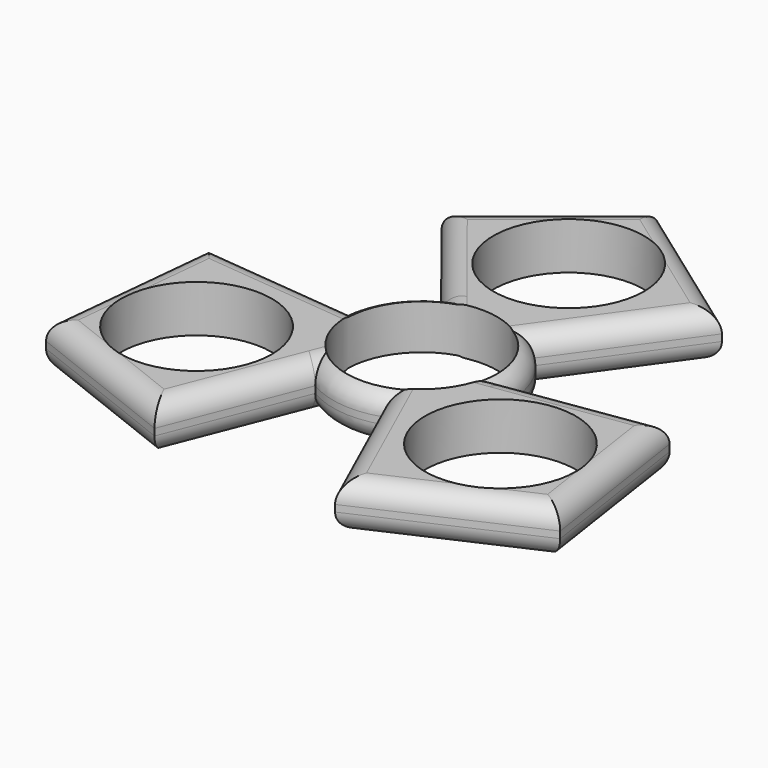
from build123d import *

# Parameters (mm, degrees)
F0_R          = 11.2
F1_DEPTH      = 7
F2_T1_DEPTH   = 41.9845753996
F2_T3_DEPTH   = 40.2947851744
F2_T5_DEPTH   = 41.9845753996
F2_T7_DEPTH   = 40.2947851744
F2_T9_DEPTH   = 41.9845753996
F2_T11_DEPTH  = 40.2947851744
F2_T16_DEPTH  = 37.6980641681
F2_S17_R      = 13.2
F2_T18_DEPTH  = 22
F2_T22_ANGLE  = 115.1707423731
F2_T28_DEPTH  = 36.5230414764
F2_S29_R      = 13.2
F2_T30_DEPTH  = 20
F2_T34_DEPTH  = 37.6980641681
F2_S35_R      = 13.2
F2_T36_DEPTH  = 22
F2_T40_ANGLE  = 115.1707423731
F2_T46_DEPTH  = 36.5230414764
F2_S47_R      = 13.2
F2_T48_DEPTH  = 21
F2_T52_DEPTH  = 36.5230414764
F2_S53_R      = 13.2
F2_T54_DEPTH  = 21
F2_T58_DEPTH  = 37.6980641681
F2_S59_R      = 13.2
F2_T60_DEPTH  = 21
F2_T64_ANGLE  = 115.1707423731
F2_T71_ANGLE  = 115.1707423731
F2_S73_R      = 11.2
F2_T74_DEPTH  = 14
F2_T77_DEPTH  = 30.1980641681
F2_S78_R      = 13.2
F2_T79_DEPTH  = 18
F2_S80_R      = 11.2
F2_T81_DEPTH  = 18
F2_T87_DEPTH  = 29.0230414764
F2_S88_R      = 13.2
F2_T89_DEPTH  = 17
F2_S90_R      = 11.2
F2_T91_DEPTH  = 17
F2_T94_ANGLE  = 115.1707423731
F2_S96_R      = 11.2
F2_T97_DEPTH  = 14
F2_T103_ANGLE = 115.1707423731
F2_S105_R     = 11.2
F2_T106_DEPTH = 15
F2_T109_DEPTH = 30.1980641681
F2_S110_R     = 13.2
F2_T111_DEPTH = 18
F2_S112_R     = 11.2
F2_T113_DEPTH = 18
F2_T119_DEPTH = 29.0230414764
F2_S120_R     = 13.2
F2_T121_DEPTH = 17
F2_S122_R     = 11.2
F2_T123_DEPTH = 17
F2_T126_ANGLE = 115.1707423731
F2_S128_R     = 11.2
F2_T129_DEPTH = 15
F2_T135_DEPTH = 29.0230414764
F2_S136_R     = 13.2
F2_T137_DEPTH = 18
F2_S138_R     = 11.2
F2_T139_DEPTH = 18
F2_T142_ANGLE = 115.1707423731
F2_S144_R     = 11.2
F2_T145_DEPTH = 14
F2_T151_DEPTH = 30.1980641681
F2_S152_R     = 13.2
F2_T153_DEPTH = 17
F2_S154_R     = 11.2
F2_T155_DEPTH = 17
F2_T158_ANGLE = 115.1707423731
F2_S160_R     = 11.2
F2_T161_DEPTH = 14
F3_T3_DEPTH   = 40.2947851744
F3_T6_DEPTH   = 41.9845753996
F3_T9_DEPTH   = 37.6980641681
F3_S10_R      = 13.2
F3_T11_DEPTH  = 22
F3_T14_DEPTH  = 36.5230414764
F3_S15_R      = 13.2
F3_T16_DEPTH  = 20
F3_T19_ANGLE  = 115.1707423731
F3_T24_DEPTH  = 40.2947851744
F3_T27_DEPTH  = 41.9845753996
F3_T30_DEPTH  = 37.6980641681
F3_S31_R      = 13.2
F3_T32_DEPTH  = 22
F3_T35_ANGLE  = 115.1707423731
F3_T40_DEPTH  = 36.5230414764
F3_S41_R      = 13.2
F3_T42_DEPTH  = 21
F3_T45_DEPTH  = 40.2947851744
F3_T48_DEPTH  = 41.9845753996
F3_T51_DEPTH  = 37.6980641681
F3_S52_R      = 13.2
F3_T53_DEPTH  = 21
F3_T56_ANGLE  = 115.1707423731
F3_T61_DEPTH  = 36.5230414764
F3_S62_R      = 13.2
F3_T63_DEPTH  = 21
F3_T67_DEPTH  = 30.1980641681
F3_S68_R      = 13.2
F3_T69_DEPTH  = 18
F3_S70_R      = 11.2
F3_T71_DEPTH  = 18
F3_T74_ANGLE  = 115.1707423731
F3_S76_R      = 11.2
F3_T77_DEPTH  = 14
F3_T82_ANGLE  = 115.1707423731
F3_S84_R      = 11.2
F3_T85_DEPTH  = 14
F3_T88_DEPTH  = 29.0230414764
F3_S89_R      = 13.2
F3_T90_DEPTH  = 17
F3_S91_R      = 11.2
F3_T92_DEPTH  = 17
F3_T97_DEPTH  = 30.1980641681
F3_S98_R      = 13.2
F3_T99_DEPTH  = 18
F3_S100_R     = 11.2
F3_T101_DEPTH = 18
F3_T104_ANGLE = 115.1707423731
F3_S106_R     = 11.2
F3_T107_DEPTH = 15
F3_T112_ANGLE = 115.1707423731
F3_S114_R     = 11.2
F3_T115_DEPTH = 15
F3_T118_DEPTH = 29.0230414764
F3_S119_R     = 13.2
F3_T120_DEPTH = 17
F3_S121_R     = 11.2
F3_T122_DEPTH = 17
F3_T127_DEPTH = 30.1980641681
F3_S128_R     = 13.2
F3_T129_DEPTH = 17
F3_S130_R     = 11.2
F3_T131_DEPTH = 17
F3_T134_ANGLE = 115.1707423731
F3_S136_R     = 11.2
F3_T137_DEPTH = 14
F3_T142_ANGLE = 115.1707423731
F3_S144_R     = 11.2
F3_T145_DEPTH = 14
F3_T148_DEPTH = 29.0230414764
F3_S149_R     = 13.2
F3_T150_DEPTH = 18
F3_S151_R     = 11.2
F3_T152_DEPTH = 18


# Not quite as in the source:
# - a fillet or chamfer that OpenCascade refuses, or shapes differently, is made with other operations: its cross-section is extruded or revolved along the edge and cut away or added


with BuildPart() as f1:
    # F0 (on Top) → F1 (new body)
    with BuildSketch(Plane.XY):
        with BuildLine():
            Line((34.4835003985, 2.9441961325), (13.1977618631, -0.2430674894))
            ThreePointArc((13.1977618631, -0.2430674894), (12.0614419071, 5.3629860267), (8.6602055702, 9.9619696588))
            Line((8.6602055702, 9.9619696588), (21.9099196474, 28.3914892903))
            Line((21.9099196474, 28.3914892903), (0, 44.1434012548))
            Line((0, 44.1434012548), (-19.7914988438, 28.3914892903))
            Line((-19.7914988438, 28.3914892903), (-6.3883783109, 11.5511307912))
            ThreePointArc((-6.3883783109, 11.5511307912), (-10.6752030928, 7.7640220844), (-12.9574215813, 2.5189731964))
            Line((-12.9574215813, 2.5189731964), (-35.5427108004, 4.7788023644))
            Line((-35.5427108004, 4.7788023644), (-38.2293068961, -22.0717006274))
            Line((-38.2293068961, -22.0717006274), (-14.6920015548, -31.3356854228))
            Line((-14.6920015548, -31.3356854228), (-6.8093835522, -11.3080633019))
            ThreePointArc((-6.8093835522, -11.3080633019), (-1.3862388143, -13.1270081111), (4.2972160111, -12.4809428552))
            Line((4.2972160111, -12.4809428552), (13.6327911529, -33.1702916547))
            Line((13.6327911529, -33.1702916547), (38.2293068961, -22.0717006274))
            Line((38.2293068961, -22.0717006274), (34.4835003985, 2.9441961325))
        make_face()
        with Locations((-23.2943706214, -12.7743324265)):
            Circle(F0_R, mode=Mode.SUBTRACT)
        Circle(F0_R, mode=Mode.SUBTRACT)
        with Locations((22.7100817084, -13.7863505101)):
            Circle(F0_R, mode=Mode.SUBTRACT)
        with Locations((0.584288913, 26.5606829366)):
            Circle(F0_R, mode=Mode.SUBTRACT)
    extrude(amount=F1_DEPTH)

    # F2: fillet of radius 3 on 15 edges, made by hand

    # F2_s2 → F2_t1 (cut)
    with BuildSketch(Plane(origin=(7.0772234014, -5.0880971618, 0), x_dir=(0, 0, 1), z_dir=(-0.8119423531, 0.5837376253, 0))):
        with BuildLine():
            ThreePointArc((4, 35.8418970888), (6.1213203436, 34.9632174324), (7, 32.8418970888))
            Line((7, 32.8418970888), (7, 35.8418970888))
            Line((7, 35.8418970888), (4, 35.8418970888))
        make_face()
    extrude(amount=F2_T1_DEPTH, mode=Mode.SUBTRACT)

    # F2_s4 → F2_t3 (cut)
    with BuildSketch(Plane(origin=(5.1814707168, -34.6037993688, 0), x_dir=(0, 0, 1), z_dir=(-0.1480861162, 0.9889744699, 0))):
        with BuildLine():
            ThreePointArc((4, 34.5392960988), (6.1213203436, 33.6606164423), (7, 31.5392960988))
            Line((7, 31.5392960988), (7, 34.5392960988))
            Line((7, 34.5392960988), (4, 34.5392960988))
        make_face()
    extrude(amount=F2_T3_DEPTH, mode=Mode.SUBTRACT)

    # F2_s6 → F2_t5 (cut)
    with BuildSketch(Plane(origin=(-7.9450330997, -3.585006673, 0), x_dir=(0, 0, 1), z_dir=(0.9115027892, 0.4112938915, 0))):
        with BuildLine():
            ThreePointArc((4, 35.8418970888), (6.1213203436, 34.9632174324), (7, 32.8418970888))
            Line((7, 32.8418970888), (7, 35.8418970888))
            Line((7, 35.8418970888), (4, 35.8418970888))
        make_face()
    extrude(amount=F2_T5_DEPTH, mode=Mode.SUBTRACT)

    # F2_s8 → F2_t7 (cut)
    with BuildSketch(Plane(origin=(-32.5585046793, 12.8146144147, 0), x_dir=(0, 0, 1), z_dir=(0.9305200728, -0.3662408964, 0))):
        with BuildLine():
            ThreePointArc((4, 34.5392960988), (6.1213203436, 33.6606164423), (7, 31.5392960988))
            Line((7, 31.5392960988), (7, 34.5392960988))
            Line((7, 34.5392960988), (4, 34.5392960988))
        make_face()
    extrude(amount=F2_T7_DEPTH, mode=Mode.SUBTRACT)

    # F2_s10 → F2_t9 (cut)
    with BuildSketch(Plane(origin=(0.8678096983, 8.6731038348, 0), x_dir=(0, 0, 1), z_dir=(-0.0995604361, -0.9950315169, 0))):
        with BuildLine():
            ThreePointArc((4, 35.8418970888), (6.1213203436, 34.9632174324), (7, 32.8418970888))
            Line((7, 32.8418970888), (7, 35.8418970888))
            Line((7, 35.8418970888), (4, 35.8418970888))
        make_face()
    extrude(amount=F2_T9_DEPTH, mode=Mode.SUBTRACT)

    # F2_s12 → F2_t11 (cut)
    with BuildSketch(Plane(origin=(27.3770339624, 21.7891849542, 0), x_dir=(0, 0, 1), z_dir=(-0.7824339565, -0.6227335736, 0))):
        with BuildLine():
            ThreePointArc((4, 34.5392960988), (6.1213203436, 33.6606164423), (7, 31.5392960988))
            Line((7, 31.5392960988), (7, 34.5392960988))
            Line((7, 34.5392960988), (4, 34.5392960988))
        make_face()
    extrude(amount=F2_T11_DEPTH, mode=Mode.SUBTRACT)


with BuildPart() as f2_tool14:
    # F2_s15 → F2_t16 (new body)
    with BuildSketch(Plane(origin=(3.294517627, 4.5824669822, 0), x_dir=(0, 0, 1), z_dir=(0.5837376253, 0.8119423531, 0))):
        with BuildLine():
            ThreePointArc((4, 1.2164111767), (6.1213203436, 0.3377315202), (7, -1.7835888233))
            Line((7, -1.7835888233), (7, 1.2164111767))
            Line((7, 1.2164111767), (4, 1.2164111767))
        make_face()
    extrude(amount=F2_T16_DEPTH)

    # F2_s17 → F2_t18 (cut, symmetric)
    with BuildSketch(Plane.XY.offset(5.5)):
        Circle(F2_S17_R)
    extrude(amount=F2_T18_DEPTH, both=True, mode=Mode.SUBTRACT)


with BuildPart() as f1_1:
    add(f1.part)

    # F2_t13: cut F2_tool14
    add(f2_tool14.part, mode=Mode.SUBTRACT)


with BuildPart() as f2_tool20:
    # F2_s21 → F2_t22 (revolve)
    with BuildSketch(Plane(origin=(0, 0, 0), x_dir=(0, 0, 1), z_dir=(-0.5535889506, -0.8327900538, 0))):
        with BuildLine():
            ThreePointArc((4, -13.2), (6.1213203436, -12.3213203436), (7, -10.2))
            Line((7, -10.2), (7, -13.2))
            Line((7, -13.2), (4, -13.2))
        make_face()
    revolve(axis=Axis((0, 0, 7), (0, 0, 1)), revolution_arc=F2_T22_ANGLE)

    split(bisect_by=Plane(origin=(0.3250183475, -2.1705940844, 0), x_dir=(0, 0, 1), z_dir=(-0.1480861162, 0.9889744699, 0)), keep=Keep.TOP)

    split(bisect_by=Plane(origin=(0.9876557531, -0.7100649717, 0), x_dir=(0, 0, 1), z_dir=(0.8119423531, -0.5837376253, 0)), keep=Keep.TOP)


with BuildPart() as f1_2:
    add(f1_1.part)

    # F2_t19: cut F2_tool20
    add(f2_tool20.part, mode=Mode.SUBTRACT)


with BuildPart() as f2_tool26:
    # F2_s27 → F2_t28 (new body)
    with BuildSketch(Plane(origin=(41.5757905756, 6.2254360887, 0), x_dir=(0, 0, 1), z_dir=(-0.9889744699, -0.1480861162, 0))):
        with BuildLine():
            ThreePointArc((4, -2.1947928388), (6.1213203436, -3.0734724953), (7, -5.1947928388))
            Line((7, -5.1947928388), (7, -2.1947928388))
            Line((7, -2.1947928388), (4, -2.1947928388))
        make_face()
    extrude(amount=F2_T28_DEPTH)

    # F2_s29 → F2_t30 (cut, symmetric)
    with BuildSketch(Plane.XY.offset(5.5)):
        Circle(F2_S29_R)
    extrude(amount=F2_T30_DEPTH, both=True, mode=Mode.SUBTRACT)


with BuildPart() as f1_3:
    add(f1_2.part)

    # F2_t25: cut F2_tool26
    add(f2_tool26.part, mode=Mode.SUBTRACT)


with BuildPart() as f2_tool32:
    # F2_s33 → F2_t34 (new body)
    with BuildSketch(Plane(origin=(2.3212740051, -5.1443694493, 0), x_dir=(0, 0, 1), z_dir=(0.4112938915, -0.9115027892, 0))):
        with BuildLine():
            ThreePointArc((4, 1.2164111767), (6.1213203436, 0.3377315202), (7, -1.7835888233))
            Line((7, -1.7835888233), (7, 1.2164111767))
            Line((7, 1.2164111767), (4, 1.2164111767))
        make_face()
    extrude(amount=F2_T34_DEPTH)

    # F2_s35 → F2_t36 (cut, symmetric)
    with BuildSketch(Plane.XY.offset(5.5)):
        Circle(F2_S35_R)
    extrude(amount=F2_T36_DEPTH, both=True, mode=Mode.SUBTRACT)


with BuildPart() as f1_4:
    add(f1_3.part)

    # F2_t31: cut F2_tool32
    add(f2_tool32.part, mode=Mode.SUBTRACT)


with BuildPart() as f2_tool38:
    # F2_s39 → F2_t40 (revolve)
    with BuildSketch(Plane(origin=(0, 0, 0), x_dir=(0, 0, 1), z_dir=(-0.4444228673, 0.8958171214, 0))):
        with BuildLine():
            ThreePointArc((4, -13.2), (6.1213203436, -12.3213203436), (7, -10.2))
            Line((7, -10.2), (7, -13.2))
            Line((7, -13.2), (4, -13.2))
        make_face()
    revolve(axis=Axis((0, 0, 7), (0, 0, 1)), revolution_arc=F2_T40_ANGLE)

    split(bisect_by=Plane(origin=(-2.0422987921, 0.8038228966, 0), x_dir=(0, 0, 1), z_dir=(0.9305200728, -0.3662408964, 0)), keep=Keep.TOP)

    split(bisect_by=Plane(origin=(-1.1087621804, -0.5003024866, 0), x_dir=(0, 0, 1), z_dir=(-0.9115027892, -0.4112938915, 0)), keep=Keep.TOP)


with BuildPart() as f1_5:
    add(f1_4.part)

    # F2_t37: cut F2_tool38
    add(f2_tool38.part, mode=Mode.SUBTRACT)


with BuildPart() as f2_tool44:
    # F2_s45 → F2_t46 (new body)
    with BuildSketch(Plane(origin=(-15.3965094853, -39.1184088652, 0), x_dir=(0, 0, 1), z_dir=(0.3662408964, 0.9305200728, 0))):
        with BuildLine():
            ThreePointArc((4, -2.1947928388), (6.1213203436, -3.0734724953), (7, -5.1947928388))
            Line((7, -5.1947928388), (7, -2.1947928388))
            Line((7, -2.1947928388), (4, -2.1947928388))
        make_face()
    extrude(amount=F2_T46_DEPTH)

    # F2_s47 → F2_t48 (cut, symmetric)
    with BuildSketch(Plane.XY.offset(5.5)):
        Circle(F2_S47_R)
    extrude(amount=F2_T48_DEPTH, both=True, mode=Mode.SUBTRACT)


with BuildPart() as f1_6:
    add(f1_5.part)

    # F2_t43: cut F2_tool44
    add(f2_tool44.part, mode=Mode.SUBTRACT)


with BuildPart() as f2_tool50:
    # F2_s51 → F2_t52 (new body)
    with BuildSketch(Plane(origin=(-26.1792810902, 32.8929727765, 0), x_dir=(0, 0, 1), z_dir=(0.6227335736, -0.7824339565, 0))):
        with BuildLine():
            ThreePointArc((4, -2.1947928388), (6.1213203436, -3.0734724953), (7, -5.1947928388))
            Line((7, -5.1947928388), (7, -2.1947928388))
            Line((7, -2.1947928388), (4, -2.1947928388))
        make_face()
    extrude(amount=F2_T52_DEPTH)

    # F2_s53 → F2_t54 (cut, symmetric)
    with BuildSketch(Plane.XY.offset(5.5)):
        Circle(F2_S53_R)
    extrude(amount=F2_T54_DEPTH, both=True, mode=Mode.SUBTRACT)


with BuildPart() as f1_7:
    add(f1_6.part)

    # F2_t49: cut F2_tool50
    add(f2_tool50.part, mode=Mode.SUBTRACT)


with BuildPart() as f2_tool56:
    # F2_s57 → F2_t58 (new body)
    with BuildSketch(Plane(origin=(-5.6157916321, 0.5619024671, 0), x_dir=(0, 0, 1), z_dir=(-0.9950315169, 0.0995604361, 0))):
        with BuildLine():
            ThreePointArc((4, 1.2164111767), (6.1213203436, 0.3377315202), (7, -1.7835888233))
            Line((7, -1.7835888233), (7, 1.2164111767))
            Line((7, 1.2164111767), (4, 1.2164111767))
        make_face()
    extrude(amount=F2_T58_DEPTH)

    # F2_s59 → F2_t60 (cut, symmetric)
    with BuildSketch(Plane.XY.offset(5.5)):
        Circle(F2_S59_R)
    extrude(amount=F2_T60_DEPTH, both=True, mode=Mode.SUBTRACT)


with BuildPart() as f1_8:
    add(f1_7.part)

    # F2_t55: cut F2_tool56
    add(f2_tool56.part, mode=Mode.SUBTRACT)


with BuildPart() as f2_tool62:
    # F2_s63 → F2_t64 (revolve)
    with BuildSketch(Plane(origin=(0, 0, 0), x_dir=(0, 0, 1), z_dir=(0.9980118179, -0.0630270676, 0))):
        with BuildLine():
            ThreePointArc((4, -13.2), (6.1213203436, -12.3213203436), (7, -10.2))
            Line((7, -10.2), (7, -13.2))
            Line((7, -13.2), (4, -13.2))
        make_face()
    revolve(axis=Axis((0, 0, 7), (0, 0, 1)), revolution_arc=F2_T64_ANGLE)

    split(bisect_by=Plane(origin=(0.1211064273, 1.2103674583, 0), x_dir=(0, 0, 1), z_dir=(0.0995604361, 0.9950315169, 0)), keep=Keep.TOP)

    split(bisect_by=Plane(origin=(1.7172804447, 1.3667711878, 0), x_dir=(0, 0, 1), z_dir=(-0.7824339565, -0.6227335736, 0)), keep=Keep.TOP)


with BuildPart() as f1_9:
    add(f1_8.part)

    # F2_t61: cut F2_tool62
    add(f2_tool62.part, mode=Mode.SUBTRACT)


with BuildPart() as f2_tool69:
    # F2_s70 → F2_t71 (revolve)
    with BuildSketch(Plane(origin=(0, 0, 0), x_dir=(0, 0, 1), z_dir=(-0.5535889506, -0.8327900538, 0))):
        with BuildLine():
            ThreePointArc((4, -13.2), (6.1213203436, -12.3213203436), (7, -10.2))
            Line((7, -10.2), (7, -13.2))
            Line((7, -13.2), (4, -13.2))
        make_face()
    revolve(axis=Axis((0, 0, 7), (0, 0, 1)), revolution_arc=F2_T71_ANGLE)

    split(bisect_by=Plane(origin=(0.9876557531, -0.7100649717, 0), x_dir=(0, 0, 1), z_dir=(-0.8119423531, 0.5837376253, 0)), keep=Keep.TOP)

    # F2_s73 → F2_t74 (cut, symmetric)
    with BuildSketch(Plane.XY.offset(5.5)):
        Circle(F2_S73_R)
    extrude(amount=F2_T74_DEPTH, both=True, mode=Mode.SUBTRACT)


with BuildPart() as f2_tool75:
    # F2_s76 → F2_t77 (new body)
    with BuildSketch(Plane(origin=(3.294517627, 4.5824669822, 0), x_dir=(0, 0, 1), z_dir=(0.5837376253, 0.8119423531, 0))):
        with BuildLine():
            ThreePointArc((4, 1.2164111767), (6.1213203436, 0.3377315202), (7, -1.7835888233))
            Line((7, -1.7835888233), (7, 1.2164111767))
            Line((7, 1.2164111767), (4, 1.2164111767))
        make_face()
    extrude(amount=F2_T77_DEPTH)

    # F2_s78 → F2_t79 (intersect, symmetric)
    with BuildSketch(Plane.XY.offset(5.5)):
        Circle(F2_S78_R)
    extrude(amount=F2_T79_DEPTH, both=True, mode=Mode.INTERSECT)

    # F2_s80 → F2_t81 (cut, symmetric)
    with BuildSketch(Plane.XY.offset(5.5)):
        Circle(F2_S80_R)
    extrude(amount=F2_T81_DEPTH, both=True, mode=Mode.SUBTRACT)


with BuildPart() as f2_tool69_1:
    add(f2_tool69.part)

    # F2_t82: intersect F2_tool75
    add(f2_tool75.part, mode=Mode.INTERSECT)


with BuildPart() as f1_10:
    add(f1_9.part)

    # F2_t67: cut F2_tool69
    add(f2_tool69_1.part, mode=Mode.SUBTRACT)


with BuildPart() as f2_tool85:
    # F2_s86 → F2_t87 (new body)
    with BuildSketch(Plane(origin=(34.1584820511, 5.1147902169, 0), x_dir=(0, 0, 1), z_dir=(-0.9889744699, -0.1480861162, 0))):
        with BuildLine():
            ThreePointArc((4, -2.1947928388), (6.1213203436, -3.0734724953), (7, -5.1947928388))
            Line((7, -5.1947928388), (7, -2.1947928388))
            Line((7, -2.1947928388), (4, -2.1947928388))
        make_face()
    extrude(amount=F2_T87_DEPTH)

    # F2_s88 → F2_t89 (intersect, symmetric)
    with BuildSketch(Plane.XY.offset(5.5)):
        Circle(F2_S88_R)
    extrude(amount=F2_T89_DEPTH, both=True, mode=Mode.INTERSECT)

    # F2_s90 → F2_t91 (cut, symmetric)
    with BuildSketch(Plane.XY.offset(5.5)):
        Circle(F2_S90_R)
    extrude(amount=F2_T91_DEPTH, both=True, mode=Mode.SUBTRACT)


with BuildPart() as f2_tool92:
    # F2_s93 → F2_t94 (revolve)
    with BuildSketch(Plane(origin=(0, 0, 0), x_dir=(0, 0, 1), z_dir=(-0.5535889506, -0.8327900538, 0))):
        with BuildLine():
            ThreePointArc((4, -13.2), (6.1213203436, -12.3213203436), (7, -10.2))
            Line((7, -10.2), (7, -13.2))
            Line((7, -13.2), (4, -13.2))
        make_face()
    revolve(axis=Axis((0, 0, 7), (0, 0, 1)), revolution_arc=F2_T94_ANGLE)

    split(bisect_by=Plane(origin=(0.3250183475, -2.1705940844, 0), x_dir=(0, 0, 1), z_dir=(0.1480861162, -0.9889744699, 0)), keep=Keep.TOP)

    # F2_s96 → F2_t97 (cut, symmetric)
    with BuildSketch(Plane.XY.offset(5.5)):
        Circle(F2_S96_R)
    extrude(amount=F2_T97_DEPTH, both=True, mode=Mode.SUBTRACT)


with BuildPart() as f2_tool85_1:
    add(f2_tool85.part)

    # F2_t98: intersect F2_tool92
    add(f2_tool92.part, mode=Mode.INTERSECT)


with BuildPart() as f1_11:
    add(f1_10.part)

    # F2_t83: cut F2_tool85
    add(f2_tool85_1.part, mode=Mode.SUBTRACT)


with BuildPart() as f2_tool101:
    # F2_s102 → F2_t103 (revolve)
    with BuildSketch(Plane(origin=(0, 0, 0), x_dir=(0, 0, 1), z_dir=(-0.4444228673, 0.8958171214, 0))):
        with BuildLine():
            ThreePointArc((4, -13.2), (6.1213203436, -12.3213203436), (7, -10.2))
            Line((7, -10.2), (7, -13.2))
            Line((7, -13.2), (4, -13.2))
        make_face()
    revolve(axis=Axis((0, 0, 7), (0, 0, 1)), revolution_arc=F2_T103_ANGLE)

    split(bisect_by=Plane(origin=(-1.1087621804, -0.5003024866, 0), x_dir=(0, 0, 1), z_dir=(0.9115027892, 0.4112938915, 0)), keep=Keep.TOP)

    # F2_s105 → F2_t106 (cut, symmetric)
    with BuildSketch(Plane.XY.offset(5.5)):
        Circle(F2_S105_R)
    extrude(amount=F2_T106_DEPTH, both=True, mode=Mode.SUBTRACT)


with BuildPart() as f2_tool107:
    # F2_s108 → F2_t109 (new body)
    with BuildSketch(Plane(origin=(2.3212740051, -5.1443694493, 0), x_dir=(0, 0, 1), z_dir=(0.4112938915, -0.9115027892, 0))):
        with BuildLine():
            ThreePointArc((4, 1.2164111767), (6.1213203436, 0.3377315202), (7, -1.7835888233))
            Line((7, -1.7835888233), (7, 1.2164111767))
            Line((7, 1.2164111767), (4, 1.2164111767))
        make_face()
    extrude(amount=F2_T109_DEPTH)

    # F2_s110 → F2_t111 (intersect, symmetric)
    with BuildSketch(Plane.XY.offset(5.5)):
        Circle(F2_S110_R)
    extrude(amount=F2_T111_DEPTH, both=True, mode=Mode.INTERSECT)

    # F2_s112 → F2_t113 (cut, symmetric)
    with BuildSketch(Plane.XY.offset(5.5)):
        Circle(F2_S112_R)
    extrude(amount=F2_T113_DEPTH, both=True, mode=Mode.SUBTRACT)


with BuildPart() as f2_tool101_1:
    add(f2_tool101.part)

    # F2_t114: intersect F2_tool107
    add(f2_tool107.part, mode=Mode.INTERSECT)


with BuildPart() as f1_12:
    add(f1_11.part)

    # F2_t99: cut F2_tool101
    add(f2_tool101_1.part, mode=Mode.SUBTRACT)


with BuildPart() as f2_tool117:
    # F2_s118 → F2_t119 (new body)
    with BuildSketch(Plane(origin=(-12.6497027627, -32.1395083194, 0), x_dir=(0, 0, 1), z_dir=(0.3662408964, 0.9305200728, 0))):
        with BuildLine():
            ThreePointArc((4, -2.1947928388), (6.1213203436, -3.0734724953), (7, -5.1947928388))
            Line((7, -5.1947928388), (7, -2.1947928388))
            Line((7, -2.1947928388), (4, -2.1947928388))
        make_face()
    extrude(amount=F2_T119_DEPTH)

    # F2_s120 → F2_t121 (intersect, symmetric)
    with BuildSketch(Plane.XY.offset(5.5)):
        Circle(F2_S120_R)
    extrude(amount=F2_T121_DEPTH, both=True, mode=Mode.INTERSECT)

    # F2_s122 → F2_t123 (cut, symmetric)
    with BuildSketch(Plane.XY.offset(5.5)):
        Circle(F2_S122_R)
    extrude(amount=F2_T123_DEPTH, both=True, mode=Mode.SUBTRACT)


with BuildPart() as f2_tool124:
    # F2_s125 → F2_t126 (revolve)
    with BuildSketch(Plane(origin=(0, 0, 0), x_dir=(0, 0, 1), z_dir=(-0.4444228673, 0.8958171214, 0))):
        with BuildLine():
            ThreePointArc((4, -13.2), (6.1213203436, -12.3213203436), (7, -10.2))
            Line((7, -10.2), (7, -13.2))
            Line((7, -13.2), (4, -13.2))
        make_face()
    revolve(axis=Axis((0, 0, 7), (0, 0, 1)), revolution_arc=F2_T126_ANGLE)

    split(bisect_by=Plane(origin=(-2.0422987921, 0.8038228966, 0), x_dir=(0, 0, 1), z_dir=(-0.9305200728, 0.3662408964, 0)), keep=Keep.TOP)

    # F2_s128 → F2_t129 (cut, symmetric)
    with BuildSketch(Plane.XY.offset(5.5)):
        Circle(F2_S128_R)
    extrude(amount=F2_T129_DEPTH, both=True, mode=Mode.SUBTRACT)


with BuildPart() as f2_tool117_1:
    add(f2_tool117.part)

    # F2_t130: intersect F2_tool124
    add(f2_tool124.part, mode=Mode.INTERSECT)


with BuildPart() as f1_13:
    add(f1_12.part)

    # F2_t115: cut F2_tool117
    add(f2_tool117_1.part, mode=Mode.SUBTRACT)


with BuildPart() as f2_tool133:
    # F2_s134 → F2_t135 (new body)
    with BuildSketch(Plane(origin=(-21.5087792884, 27.0247181025, 0), x_dir=(0, 0, 1), z_dir=(0.6227335736, -0.7824339565, 0))):
        with BuildLine():
            ThreePointArc((4, -2.1947928388), (6.1213203436, -3.0734724953), (7, -5.1947928388))
            Line((7, -5.1947928388), (7, -2.1947928388))
            Line((7, -2.1947928388), (4, -2.1947928388))
        make_face()
    extrude(amount=F2_T135_DEPTH)

    # F2_s136 → F2_t137 (intersect, symmetric)
    with BuildSketch(Plane.XY.offset(5.5)):
        Circle(F2_S136_R)
    extrude(amount=F2_T137_DEPTH, both=True, mode=Mode.INTERSECT)

    # F2_s138 → F2_t139 (cut, symmetric)
    with BuildSketch(Plane.XY.offset(5.5)):
        Circle(F2_S138_R)
    extrude(amount=F2_T139_DEPTH, both=True, mode=Mode.SUBTRACT)


with BuildPart() as f2_tool140:
    # F2_s141 → F2_t142 (revolve)
    with BuildSketch(Plane(origin=(0, 0, 0), x_dir=(0, 0, 1), z_dir=(0.9980118179, -0.0630270676, 0))):
        with BuildLine():
            ThreePointArc((4, -13.2), (6.1213203436, -12.3213203436), (7, -10.2))
            Line((7, -10.2), (7, -13.2))
            Line((7, -13.2), (4, -13.2))
        make_face()
    revolve(axis=Axis((0, 0, 7), (0, 0, 1)), revolution_arc=F2_T142_ANGLE)

    split(bisect_by=Plane(origin=(1.7172804447, 1.3667711878, 0), x_dir=(0, 0, 1), z_dir=(0.7824339565, 0.6227335736, 0)), keep=Keep.TOP)

    # F2_s144 → F2_t145 (cut, symmetric)
    with BuildSketch(Plane.XY.offset(5.5)):
        Circle(F2_S144_R)
    extrude(amount=F2_T145_DEPTH, both=True, mode=Mode.SUBTRACT)


with BuildPart() as f2_tool133_1:
    add(f2_tool133.part)

    # F2_t146: intersect F2_tool140
    add(f2_tool140.part, mode=Mode.INTERSECT)


with BuildPart() as f1_14:
    add(f1_13.part)

    # F2_t131: cut F2_tool133
    add(f2_tool133_1.part, mode=Mode.SUBTRACT)


with BuildPart() as f2_tool149:
    # F2_s150 → F2_t151 (new body)
    with BuildSketch(Plane(origin=(-5.6157916321, 0.5619024671, 0), x_dir=(0, 0, 1), z_dir=(-0.9950315169, 0.0995604361, 0))):
        with BuildLine():
            ThreePointArc((4, 1.2164111767), (6.1213203436, 0.3377315202), (7, -1.7835888233))
            Line((7, -1.7835888233), (7, 1.2164111767))
            Line((7, 1.2164111767), (4, 1.2164111767))
        make_face()
    extrude(amount=F2_T151_DEPTH)

    # F2_s152 → F2_t153 (intersect, symmetric)
    with BuildSketch(Plane.XY.offset(5.5)):
        Circle(F2_S152_R)
    extrude(amount=F2_T153_DEPTH, both=True, mode=Mode.INTERSECT)

    # F2_s154 → F2_t155 (cut, symmetric)
    with BuildSketch(Plane.XY.offset(5.5)):
        Circle(F2_S154_R)
    extrude(amount=F2_T155_DEPTH, both=True, mode=Mode.SUBTRACT)


with BuildPart() as f2_tool156:
    # F2_s157 → F2_t158 (revolve)
    with BuildSketch(Plane(origin=(0, 0, 0), x_dir=(0, 0, 1), z_dir=(0.9980118179, -0.0630270676, 0))):
        with BuildLine():
            ThreePointArc((4, -13.2), (6.1213203436, -12.3213203436), (7, -10.2))
            Line((7, -10.2), (7, -13.2))
            Line((7, -13.2), (4, -13.2))
        make_face()
    revolve(axis=Axis((0, 0, 7), (0, 0, 1)), revolution_arc=F2_T158_ANGLE)

    split(bisect_by=Plane(origin=(0.1211064273, 1.2103674583, 0), x_dir=(0, 0, 1), z_dir=(-0.0995604361, -0.9950315169, 0)), keep=Keep.TOP)

    # F2_s160 → F2_t161 (cut, symmetric)
    with BuildSketch(Plane.XY.offset(5.5)):
        Circle(F2_S160_R)
    extrude(amount=F2_T161_DEPTH, both=True, mode=Mode.SUBTRACT)


with BuildPart() as f2_tool149_1:
    add(f2_tool149.part)

    # F2_t162: intersect F2_tool156
    add(f2_tool156.part, mode=Mode.INTERSECT)


with BuildPart() as f1_15:
    add(f1_14.part)

    # F2_t147: cut F2_tool149
    add(f2_tool149_1.part, mode=Mode.SUBTRACT)

    # F3: fillet of radius 3 on 15 edges, made by hand


with BuildPart() as f3_tool1:
    # F3_s2 → F3_t3 (new body)
    with BuildSketch(Plane(origin=(27.3770339624, 21.7891849542, 0), x_dir=(0, 0, 1), z_dir=(-0.7824339565, -0.6227335736, 0))):
        with BuildLine():
            ThreePointArc((3, 34.5392960988), (0.8786796564, 33.6606164423), (0, 31.5392960988))
            Line((0, 31.5392960988), (0, 34.5392960988))
            Line((0, 34.5392960988), (3, 34.5392960988))
        make_face()
    extrude(amount=F3_T3_DEPTH)


with BuildPart() as f3_tool4:
    # F3_s5 → F3_t6 (new body)
    with BuildSketch(Plane(origin=(7.0772234014, -5.0880971618, 0), x_dir=(0, 0, 1), z_dir=(-0.8119423531, 0.5837376253, 0))):
        with BuildLine():
            ThreePointArc((3, 35.8418970888), (0.8786796564, 34.9632174324), (0, 32.8418970888))
            Line((0, 32.8418970888), (0, 35.8418970888))
            Line((0, 35.8418970888), (3, 35.8418970888))
        make_face()
    extrude(amount=F3_T6_DEPTH)


with BuildPart() as f3_tool7:
    # F3_s8 → F3_t9 (new body)
    with BuildSketch(Plane(origin=(3.294517627, 4.5824669822, 0), x_dir=(0, 0, 1), z_dir=(0.5837376253, 0.8119423531, 0))):
        with BuildLine():
            ThreePointArc((3, 1.2164111767), (0.8786796564, 0.3377315202), (0, -1.7835888233))
            Line((0, -1.7835888233), (0, 1.2164111767))
            Line((0, 1.2164111767), (3, 1.2164111767))
        make_face()
    extrude(amount=F3_T9_DEPTH)

    # F3_s10 → F3_t11 (cut, symmetric)
    with BuildSketch(Plane.XY.offset(1.5)):
        Circle(F3_S10_R)
    extrude(amount=F3_T11_DEPTH, both=True, mode=Mode.SUBTRACT)


with BuildPart() as f3_tool12:
    # F3_s13 → F3_t14 (new body)
    with BuildSketch(Plane(origin=(41.5757905756, 6.2254360887, 0), x_dir=(0, 0, 1), z_dir=(-0.9889744699, -0.1480861162, 0))):
        with BuildLine():
            ThreePointArc((3, -2.1947928388), (0.8786796564, -3.0734724953), (0, -5.1947928388))
            Line((0, -5.1947928388), (0, -2.1947928388))
            Line((0, -2.1947928388), (3, -2.1947928388))
        make_face()
    extrude(amount=F3_T14_DEPTH)

    # F3_s15 → F3_t16 (cut, symmetric)
    with BuildSketch(Plane.XY.offset(1.5)):
        Circle(F3_S15_R)
    extrude(amount=F3_T16_DEPTH, both=True, mode=Mode.SUBTRACT)


with BuildPart() as f3_tool17:
    # F3_s18 → F3_t19 (revolve)
    with BuildSketch(Plane(origin=(0, 0, 0), x_dir=(0, 0, 1), z_dir=(-0.5535889506, -0.8327900538, 0))):
        with BuildLine():
            ThreePointArc((3, -13.2), (0.8786796564, -12.3213203436), (0, -10.2))
            Line((0, -10.2), (0, -13.2))
            Line((0, -13.2), (3, -13.2))
        make_face()
    revolve(axis=Axis((0, 0, 0), (0, 0, 1)), revolution_arc=F3_T19_ANGLE)

    split(bisect_by=Plane(origin=(0.9876557531, -0.7100649717, 0), x_dir=(0, 0, 1), z_dir=(0.8119423531, -0.5837376253, 0)), keep=Keep.TOP)

    split(bisect_by=Plane(origin=(0.3250183475, -2.1705940844, 0), x_dir=(0, 0, 1), z_dir=(-0.1480861162, 0.9889744699, 0)), keep=Keep.TOP)


with BuildPart() as f3_tool22:
    # F3_s23 → F3_t24 (new body)
    with BuildSketch(Plane(origin=(5.1814707168, -34.6037993688, 0), x_dir=(0, 0, 1), z_dir=(-0.1480861162, 0.9889744699, 0))):
        with BuildLine():
            ThreePointArc((3, 34.5392960988), (0.8786796564, 33.6606164423), (0, 31.5392960988))
            Line((0, 31.5392960988), (0, 34.5392960988))
            Line((0, 34.5392960988), (3, 34.5392960988))
        make_face()
    extrude(amount=F3_T24_DEPTH)


with BuildPart() as f3_tool25:
    # F3_s26 → F3_t27 (new body)
    with BuildSketch(Plane(origin=(-7.9450330997, -3.585006673, 0), x_dir=(0, 0, 1), z_dir=(0.9115027892, 0.4112938915, 0))):
        with BuildLine():
            ThreePointArc((3, 35.8418970888), (0.8786796564, 34.9632174324), (0, 32.8418970888))
            Line((0, 32.8418970888), (0, 35.8418970888))
            Line((0, 35.8418970888), (3, 35.8418970888))
        make_face()
    extrude(amount=F3_T27_DEPTH)


with BuildPart() as f3_tool28:
    # F3_s29 → F3_t30 (new body)
    with BuildSketch(Plane(origin=(2.3212740051, -5.1443694493, 0), x_dir=(0, 0, 1), z_dir=(0.4112938915, -0.9115027892, 0))):
        with BuildLine():
            ThreePointArc((3, 1.2164111767), (0.8786796564, 0.3377315202), (0, -1.7835888233))
            Line((0, -1.7835888233), (0, 1.2164111767))
            Line((0, 1.2164111767), (3, 1.2164111767))
        make_face()
    extrude(amount=F3_T30_DEPTH)

    # F3_s31 → F3_t32 (cut, symmetric)
    with BuildSketch(Plane.XY.offset(1.5)):
        Circle(F3_S31_R)
    extrude(amount=F3_T32_DEPTH, both=True, mode=Mode.SUBTRACT)


with BuildPart() as f3_tool33:
    # F3_s34 → F3_t35 (revolve)
    with BuildSketch(Plane(origin=(0, 0, 0), x_dir=(0, 0, 1), z_dir=(-0.4444228673, 0.8958171214, 0))):
        with BuildLine():
            ThreePointArc((3, -13.2), (0.8786796564, -12.3213203436), (0, -10.2))
            Line((0, -10.2), (0, -13.2))
            Line((0, -13.2), (3, -13.2))
        make_face()
    revolve(axis=Axis((0, 0, 0), (0, 0, 1)), revolution_arc=F3_T35_ANGLE)

    split(bisect_by=Plane(origin=(-1.1087621804, -0.5003024866, 0), x_dir=(0, 0, 1), z_dir=(-0.9115027892, -0.4112938915, 0)), keep=Keep.TOP)

    split(bisect_by=Plane(origin=(-2.0422987921, 0.8038228966, 0), x_dir=(0, 0, 1), z_dir=(0.9305200728, -0.3662408964, 0)), keep=Keep.TOP)


with BuildPart() as f3_tool38:
    # F3_s39 → F3_t40 (new body)
    with BuildSketch(Plane(origin=(-15.3965094853, -39.1184088652, 0), x_dir=(0, 0, 1), z_dir=(0.3662408964, 0.9305200728, 0))):
        with BuildLine():
            ThreePointArc((3, -2.1947928388), (0.8786796564, -3.0734724953), (0, -5.1947928388))
            Line((0, -5.1947928388), (0, -2.1947928388))
            Line((0, -2.1947928388), (3, -2.1947928388))
        make_face()
    extrude(amount=F3_T40_DEPTH)

    # F3_s41 → F3_t42 (cut, symmetric)
    with BuildSketch(Plane.XY.offset(1.5)):
        Circle(F3_S41_R)
    extrude(amount=F3_T42_DEPTH, both=True, mode=Mode.SUBTRACT)


with BuildPart() as f3_tool43:
    # F3_s44 → F3_t45 (new body)
    with BuildSketch(Plane(origin=(-32.5585046793, 12.8146144147, 0), x_dir=(0, 0, 1), z_dir=(0.9305200728, -0.3662408964, 0))):
        with BuildLine():
            ThreePointArc((3, 34.5392960988), (0.8786796564, 33.6606164423), (0, 31.5392960988))
            Line((0, 31.5392960988), (0, 34.5392960988))
            Line((0, 34.5392960988), (3, 34.5392960988))
        make_face()
    extrude(amount=F3_T45_DEPTH)


with BuildPart() as f3_tool46:
    # F3_s47 → F3_t48 (new body)
    with BuildSketch(Plane(origin=(0.8678096983, 8.6731038348, 0), x_dir=(0, 0, 1), z_dir=(-0.0995604361, -0.9950315169, 0))):
        with BuildLine():
            ThreePointArc((3, 35.8418970888), (0.8786796564, 34.9632174324), (0, 32.8418970888))
            Line((0, 32.8418970888), (0, 35.8418970888))
            Line((0, 35.8418970888), (3, 35.8418970888))
        make_face()
    extrude(amount=F3_T48_DEPTH)


with BuildPart() as f3_tool49:
    # F3_s50 → F3_t51 (new body)
    with BuildSketch(Plane(origin=(-5.6157916321, 0.5619024671, 0), x_dir=(0, 0, 1), z_dir=(-0.9950315169, 0.0995604361, 0))):
        with BuildLine():
            ThreePointArc((3, 1.2164111767), (0.8786796564, 0.3377315202), (0, -1.7835888233))
            Line((0, -1.7835888233), (0, 1.2164111767))
            Line((0, 1.2164111767), (3, 1.2164111767))
        make_face()
    extrude(amount=F3_T51_DEPTH)

    # F3_s52 → F3_t53 (cut, symmetric)
    with BuildSketch(Plane.XY.offset(1.5)):
        Circle(F3_S52_R)
    extrude(amount=F3_T53_DEPTH, both=True, mode=Mode.SUBTRACT)


with BuildPart() as f3_tool54:
    # F3_s55 → F3_t56 (revolve)
    with BuildSketch(Plane(origin=(0, 0, 0), x_dir=(0, 0, 1), z_dir=(0.9980118179, -0.0630270676, 0))):
        with BuildLine():
            ThreePointArc((3, -13.2), (0.8786796564, -12.3213203436), (0, -10.2))
            Line((0, -10.2), (0, -13.2))
            Line((0, -13.2), (3, -13.2))
        make_face()
    revolve(axis=Axis((0, 0, 0), (0, 0, 1)), revolution_arc=F3_T56_ANGLE)

    split(bisect_by=Plane(origin=(0.1211064273, 1.2103674583, 0), x_dir=(0, 0, 1), z_dir=(0.0995604361, 0.9950315169, 0)), keep=Keep.TOP)

    split(bisect_by=Plane(origin=(1.7172804447, 1.3667711878, 0), x_dir=(0, 0, 1), z_dir=(-0.7824339565, -0.6227335736, 0)), keep=Keep.TOP)


with BuildPart() as f3_tool59:
    # F3_s60 → F3_t61 (new body)
    with BuildSketch(Plane(origin=(-26.1792810902, 32.8929727765, 0), x_dir=(0, 0, 1), z_dir=(0.6227335736, -0.7824339565, 0))):
        with BuildLine():
            ThreePointArc((3, -2.1947928388), (0.8786796564, -3.0734724953), (0, -5.1947928388))
            Line((0, -5.1947928388), (0, -2.1947928388))
            Line((0, -2.1947928388), (3, -2.1947928388))
        make_face()
    extrude(amount=F3_T61_DEPTH)

    # F3_s62 → F3_t63 (cut, symmetric)
    with BuildSketch(Plane.XY.offset(1.5)):
        Circle(F3_S62_R)
    extrude(amount=F3_T63_DEPTH, both=True, mode=Mode.SUBTRACT)


with BuildPart() as f3_tool65:
    # F3_s66 → F3_t67 (new body)
    with BuildSketch(Plane(origin=(3.294517627, 4.5824669822, 0), x_dir=(0, 0, 1), z_dir=(0.5837376253, 0.8119423531, 0))):
        with BuildLine():
            ThreePointArc((3, 1.2164111767), (0.8786796564, 0.3377315202), (0, -1.7835888233))
            Line((0, -1.7835888233), (0, 1.2164111767))
            Line((0, 1.2164111767), (3, 1.2164111767))
        make_face()
    extrude(amount=F3_T67_DEPTH)

    # F3_s68 → F3_t69 (intersect, symmetric)
    with BuildSketch(Plane.XY.offset(1.5)):
        Circle(F3_S68_R)
    extrude(amount=F3_T69_DEPTH, both=True, mode=Mode.INTERSECT)

    # F3_s70 → F3_t71 (cut, symmetric)
    with BuildSketch(Plane.XY.offset(1.5)):
        Circle(F3_S70_R)
    extrude(amount=F3_T71_DEPTH, both=True, mode=Mode.SUBTRACT)


with BuildPart() as f3_tool72:
    # F3_s73 → F3_t74 (revolve)
    with BuildSketch(Plane(origin=(0, 0, 0), x_dir=(0, 0, 1), z_dir=(-0.5535889506, -0.8327900538, 0))):
        with BuildLine():
            ThreePointArc((3, -13.2), (0.8786796564, -12.3213203436), (0, -10.2))
            Line((0, -10.2), (0, -13.2))
            Line((0, -13.2), (3, -13.2))
        make_face()
    revolve(axis=Axis((0, 0, 0), (0, 0, 1)), revolution_arc=F3_T74_ANGLE)

    split(bisect_by=Plane(origin=(0.9876557531, -0.7100649717, 0), x_dir=(0, 0, 1), z_dir=(-0.8119423531, 0.5837376253, 0)), keep=Keep.TOP)

    # F3_s76 → F3_t77 (cut, symmetric)
    with BuildSketch(Plane.XY.offset(1.5)):
        Circle(F3_S76_R)
    extrude(amount=F3_T77_DEPTH, both=True, mode=Mode.SUBTRACT)


with BuildPart() as f3_tool65_1:
    add(f3_tool65.part)

    # F3_t78: intersect F3_tool72
    add(f3_tool72.part, mode=Mode.INTERSECT)


with BuildPart() as f3_tool80:
    # F3_s81 → F3_t82 (revolve)
    with BuildSketch(Plane(origin=(0, 0, 0), x_dir=(0, 0, 1), z_dir=(-0.5535889506, -0.8327900538, 0))):
        with BuildLine():
            ThreePointArc((3, -13.2), (0.8786796564, -12.3213203436), (0, -10.2))
            Line((0, -10.2), (0, -13.2))
            Line((0, -13.2), (3, -13.2))
        make_face()
    revolve(axis=Axis((0, 0, 0), (0, 0, 1)), revolution_arc=F3_T82_ANGLE)

    split(bisect_by=Plane(origin=(0.3250183475, -2.1705940844, 0), x_dir=(0, 0, 1), z_dir=(0.1480861162, -0.9889744699, 0)), keep=Keep.TOP)

    # F3_s84 → F3_t85 (cut, symmetric)
    with BuildSketch(Plane.XY.offset(1.5)):
        Circle(F3_S84_R)
    extrude(amount=F3_T85_DEPTH, both=True, mode=Mode.SUBTRACT)


with BuildPart() as f3_tool86:
    # F3_s87 → F3_t88 (new body)
    with BuildSketch(Plane(origin=(34.1584820511, 5.1147902169, 0), x_dir=(0, 0, 1), z_dir=(-0.9889744699, -0.1480861162, 0))):
        with BuildLine():
            ThreePointArc((3, -2.1947928388), (0.8786796564, -3.0734724953), (0, -5.1947928388))
            Line((0, -5.1947928388), (0, -2.1947928388))
            Line((0, -2.1947928388), (3, -2.1947928388))
        make_face()
    extrude(amount=F3_T88_DEPTH)

    # F3_s89 → F3_t90 (intersect, symmetric)
    with BuildSketch(Plane.XY.offset(1.5)):
        Circle(F3_S89_R)
    extrude(amount=F3_T90_DEPTH, both=True, mode=Mode.INTERSECT)

    # F3_s91 → F3_t92 (cut, symmetric)
    with BuildSketch(Plane.XY.offset(1.5)):
        Circle(F3_S91_R)
    extrude(amount=F3_T92_DEPTH, both=True, mode=Mode.SUBTRACT)


with BuildPart() as f3_tool80_1:
    add(f3_tool80.part)

    # F3_t93: intersect F3_tool86
    add(f3_tool86.part, mode=Mode.INTERSECT)


with BuildPart() as f3_tool95:
    # F3_s96 → F3_t97 (new body)
    with BuildSketch(Plane(origin=(2.3212740051, -5.1443694493, 0), x_dir=(0, 0, 1), z_dir=(0.4112938915, -0.9115027892, 0))):
        with BuildLine():
            ThreePointArc((3, 1.2164111767), (0.8786796564, 0.3377315202), (0, -1.7835888233))
            Line((0, -1.7835888233), (0, 1.2164111767))
            Line((0, 1.2164111767), (3, 1.2164111767))
        make_face()
    extrude(amount=F3_T97_DEPTH)

    # F3_s98 → F3_t99 (intersect, symmetric)
    with BuildSketch(Plane.XY.offset(1.5)):
        Circle(F3_S98_R)
    extrude(amount=F3_T99_DEPTH, both=True, mode=Mode.INTERSECT)

    # F3_s100 → F3_t101 (cut, symmetric)
    with BuildSketch(Plane.XY.offset(1.5)):
        Circle(F3_S100_R)
    extrude(amount=F3_T101_DEPTH, both=True, mode=Mode.SUBTRACT)


with BuildPart() as f3_tool102:
    # F3_s103 → F3_t104 (revolve)
    with BuildSketch(Plane(origin=(0, 0, 0), x_dir=(0, 0, 1), z_dir=(-0.4444228673, 0.8958171214, 0))):
        with BuildLine():
            ThreePointArc((3, -13.2), (0.8786796564, -12.3213203436), (0, -10.2))
            Line((0, -10.2), (0, -13.2))
            Line((0, -13.2), (3, -13.2))
        make_face()
    revolve(axis=Axis((0, 0, 0), (0, 0, 1)), revolution_arc=F3_T104_ANGLE)

    split(bisect_by=Plane(origin=(-1.1087621804, -0.5003024866, 0), x_dir=(0, 0, 1), z_dir=(0.9115027892, 0.4112938915, 0)), keep=Keep.TOP)

    # F3_s106 → F3_t107 (cut, symmetric)
    with BuildSketch(Plane.XY.offset(1.5)):
        Circle(F3_S106_R)
    extrude(amount=F3_T107_DEPTH, both=True, mode=Mode.SUBTRACT)


with BuildPart() as f3_tool95_1:
    add(f3_tool95.part)

    # F3_t108: intersect F3_tool102
    add(f3_tool102.part, mode=Mode.INTERSECT)


with BuildPart() as f3_tool110:
    # F3_s111 → F3_t112 (revolve)
    with BuildSketch(Plane(origin=(0, 0, 0), x_dir=(0, 0, 1), z_dir=(-0.4444228673, 0.8958171214, 0))):
        with BuildLine():
            ThreePointArc((3, -13.2), (0.8786796564, -12.3213203436), (0, -10.2))
            Line((0, -10.2), (0, -13.2))
            Line((0, -13.2), (3, -13.2))
        make_face()
    revolve(axis=Axis((0, 0, 0), (0, 0, 1)), revolution_arc=F3_T112_ANGLE)

    split(bisect_by=Plane(origin=(-2.0422987921, 0.8038228966, 0), x_dir=(0, 0, 1), z_dir=(-0.9305200728, 0.3662408964, 0)), keep=Keep.TOP)

    # F3_s114 → F3_t115 (cut, symmetric)
    with BuildSketch(Plane.XY.offset(1.5)):
        Circle(F3_S114_R)
    extrude(amount=F3_T115_DEPTH, both=True, mode=Mode.SUBTRACT)


with BuildPart() as f3_tool116:
    # F3_s117 → F3_t118 (new body)
    with BuildSketch(Plane(origin=(-12.6497027627, -32.1395083194, 0), x_dir=(0, 0, 1), z_dir=(0.3662408964, 0.9305200728, 0))):
        with BuildLine():
            ThreePointArc((3, -2.1947928388), (0.8786796564, -3.0734724953), (0, -5.1947928388))
            Line((0, -5.1947928388), (0, -2.1947928388))
            Line((0, -2.1947928388), (3, -2.1947928388))
        make_face()
    extrude(amount=F3_T118_DEPTH)

    # F3_s119 → F3_t120 (intersect, symmetric)
    with BuildSketch(Plane.XY.offset(1.5)):
        Circle(F3_S119_R)
    extrude(amount=F3_T120_DEPTH, both=True, mode=Mode.INTERSECT)

    # F3_s121 → F3_t122 (cut, symmetric)
    with BuildSketch(Plane.XY.offset(1.5)):
        Circle(F3_S121_R)
    extrude(amount=F3_T122_DEPTH, both=True, mode=Mode.SUBTRACT)


with BuildPart() as f3_tool110_1:
    add(f3_tool110.part)

    # F3_t123: intersect F3_tool116
    add(f3_tool116.part, mode=Mode.INTERSECT)


with BuildPart() as f3_tool125:
    # F3_s126 → F3_t127 (new body)
    with BuildSketch(Plane(origin=(-5.6157916321, 0.5619024671, 0), x_dir=(0, 0, 1), z_dir=(-0.9950315169, 0.0995604361, 0))):
        with BuildLine():
            ThreePointArc((3, 1.2164111767), (0.8786796564, 0.3377315202), (0, -1.7835888233))
            Line((0, -1.7835888233), (0, 1.2164111767))
            Line((0, 1.2164111767), (3, 1.2164111767))
        make_face()
    extrude(amount=F3_T127_DEPTH)

    # F3_s128 → F3_t129 (intersect, symmetric)
    with BuildSketch(Plane.XY.offset(1.5)):
        Circle(F3_S128_R)
    extrude(amount=F3_T129_DEPTH, both=True, mode=Mode.INTERSECT)

    # F3_s130 → F3_t131 (cut, symmetric)
    with BuildSketch(Plane.XY.offset(1.5)):
        Circle(F3_S130_R)
    extrude(amount=F3_T131_DEPTH, both=True, mode=Mode.SUBTRACT)


with BuildPart() as f3_tool132:
    # F3_s133 → F3_t134 (revolve)
    with BuildSketch(Plane(origin=(0, 0, 0), x_dir=(0, 0, 1), z_dir=(0.9980118179, -0.0630270676, 0))):
        with BuildLine():
            ThreePointArc((3, -13.2), (0.8786796564, -12.3213203436), (0, -10.2))
            Line((0, -10.2), (0, -13.2))
            Line((0, -13.2), (3, -13.2))
        make_face()
    revolve(axis=Axis((0, 0, 0), (0, 0, 1)), revolution_arc=F3_T134_ANGLE)

    split(bisect_by=Plane(origin=(0.1211064273, 1.2103674583, 0), x_dir=(0, 0, 1), z_dir=(-0.0995604361, -0.9950315169, 0)), keep=Keep.TOP)

    # F3_s136 → F3_t137 (cut, symmetric)
    with BuildSketch(Plane.XY.offset(1.5)):
        Circle(F3_S136_R)
    extrude(amount=F3_T137_DEPTH, both=True, mode=Mode.SUBTRACT)


with BuildPart() as f3_tool125_1:
    add(f3_tool125.part)

    # F3_t138: intersect F3_tool132
    add(f3_tool132.part, mode=Mode.INTERSECT)


with BuildPart() as f3_tool140:
    # F3_s141 → F3_t142 (revolve)
    with BuildSketch(Plane(origin=(0, 0, 0), x_dir=(0, 0, 1), z_dir=(0.9980118179, -0.0630270676, 0))):
        with BuildLine():
            ThreePointArc((3, -13.2), (0.8786796564, -12.3213203436), (0, -10.2))
            Line((0, -10.2), (0, -13.2))
            Line((0, -13.2), (3, -13.2))
        make_face()
    revolve(axis=Axis((0, 0, 0), (0, 0, 1)), revolution_arc=F3_T142_ANGLE)

    split(bisect_by=Plane(origin=(1.7172804447, 1.3667711878, 0), x_dir=(0, 0, 1), z_dir=(0.7824339565, 0.6227335736, 0)), keep=Keep.TOP)

    # F3_s144 → F3_t145 (cut, symmetric)
    with BuildSketch(Plane.XY.offset(1.5)):
        Circle(F3_S144_R)
    extrude(amount=F3_T145_DEPTH, both=True, mode=Mode.SUBTRACT)


with BuildPart() as f3_tool146:
    # F3_s147 → F3_t148 (new body)
    with BuildSketch(Plane(origin=(-21.5087792884, 27.0247181025, 0), x_dir=(0, 0, 1), z_dir=(0.6227335736, -0.7824339565, 0))):
        with BuildLine():
            ThreePointArc((3, -2.1947928388), (0.8786796564, -3.0734724953), (0, -5.1947928388))
            Line((0, -5.1947928388), (0, -2.1947928388))
            Line((0, -2.1947928388), (3, -2.1947928388))
        make_face()
    extrude(amount=F3_T148_DEPTH)

    # F3_s149 → F3_t150 (intersect, symmetric)
    with BuildSketch(Plane.XY.offset(1.5)):
        Circle(F3_S149_R)
    extrude(amount=F3_T150_DEPTH, both=True, mode=Mode.INTERSECT)

    # F3_s151 → F3_t152 (cut, symmetric)
    with BuildSketch(Plane.XY.offset(1.5)):
        Circle(F3_S151_R)
    extrude(amount=F3_T152_DEPTH, both=True, mode=Mode.SUBTRACT)


with BuildPart() as f3_tool140_1:
    add(f3_tool140.part)

    # F3_t153: intersect F3_tool146
    add(f3_tool146.part, mode=Mode.INTERSECT)


with BuildPart() as f1_16:
    add(f1_15.part)

    # F3_t154: cut F3_tool1, F3_tool4, F3_tool7, F3_tool12, F3_tool17, F3_tool22, F3_tool25, F3_tool28, F3_tool33, F3_tool38, F3_tool43, F3_tool46, F3_tool49, F3_tool54, F3_tool59, F3_tool65, F3_tool80, F3_tool95, F3_tool110, F3_tool125, F3_tool140
    add([f3_tool1.part, f3_tool4.part, f3_tool7.part, f3_tool12.part, f3_tool17.part, f3_tool22.part, f3_tool25.part, f3_tool28.part, f3_tool33.part, f3_tool38.part, f3_tool43.part, f3_tool46.part, f3_tool49.part, f3_tool54.part, f3_tool59.part, f3_tool65_1.part, f3_tool80_1.part, f3_tool95_1.part, f3_tool110_1.part, f3_tool125_1.part, f3_tool140_1.part], mode=Mode.SUBTRACT)


solid = f1_16.part
